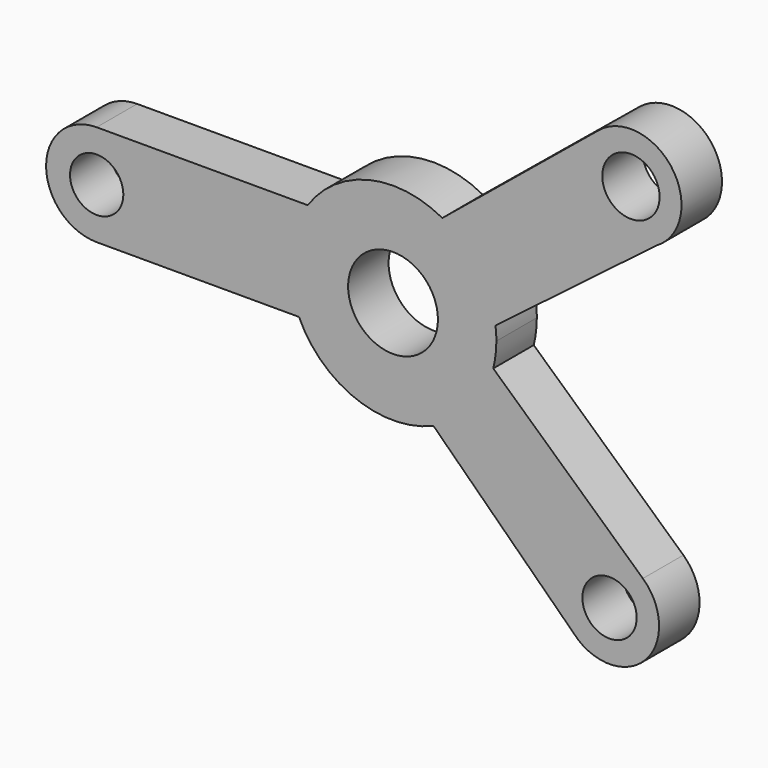
from build123d import *

# Parameters (mm, degrees)
F1_DEPTH  = 25.4
F2_R      = 22.5453784596
F3_DEPTH  = 25.401
F4_R      = 15.5169822629
F4_R_2    = 14.6151483758
F4_R_3    = 13.5851891759
F5_DEPTH  = 419
F6_R      = 14.3828522328
F7_DEPTH  = 25.401
F8_R      = 13.6217726984
F9_DEPTH  = 25.4
F10_R     = 13.3826357349
F11_DEPTH = 25.4


# Not quite as in the source:
# - an extrude ends at something that could not be found from the text; its depth is read off the source's solid


with BuildPart() as f1:
    # F0 (on Front) → F1 (new body)
    with BuildSketch(Plane.XZ):
        with BuildLine():
            ThreePointArc((50.3233435561, -12.5877974986), (51.4847298632, -6.3414622483), (51.873804107, 0))
            ThreePointArc((51.873804107, 0), (51.7629612184, 3.3893064834), (51.4309062461, 6.7641285647))
            ThreePointArc((51.4309062461, 6.7641285647), (42.7546046022, 29.3757610599), (24.7585971482, 45.5840259278))
            ThreePointArc((24.7585971482, 45.5840259278), (-12.1730496974, 50.4252755431), (-42.8284505735, 29.2679923125))
            ThreePointArc((-42.8284505735, 29.2679923125), (-51.683323237, 4.4413569672), (-47.1939000029, -21.5320076875))
            ThreePointArc((-47.1939000029, -21.5320076875), (-18.7719046051, -48.3581135905), (20.3057196076, -47.7343618764))
            ThreePointArc((20.3057196076, -47.7343618764), (39.4453595209, -33.6890956364), (50.3233435561, -12.5877974986))
        make_face()
        with BuildLine():
            ThreePointArc((24.7585971482, 45.5840259278), (42.7546046022, 29.3757610599), (51.4309062461, 6.7641285647))
            Line((51.4309062461, 6.7641285647), (132.2230654066, 68.3692177878))
            ThreePointArc((132.2230654066, 68.3692177878), (140.3155469651, 104.8046621717), (103.3515533001, 109.9711926872))
            Line((103.3515533001, 109.9711926872), (24.7585971482, 45.5840259278))
        make_face()
        with BuildLine():
            Line((125.4517560768, -80.9857626154), (50.3233435561, -12.5877974986))
            ThreePointArc((50.3233435561, -12.5877974986), (39.4453595209, -33.6890956364), (20.3057196076, -47.7343618764))
            Line((20.3057196076, -47.7343618764), (93.0013113713, -118.7126045859))
            ThreePointArc((93.0013113713, -118.7126045859), (127.5656184462, -115.6234022642), (125.4517560768, -80.9857626154))
        make_face()
        with BuildLine():
            ThreePointArc((-47.1939000029, -21.5320076875), (-51.683323237, 4.4413569672), (-42.8284505735, 29.2679923125))
            Line((-42.8284505735, 29.2679923125), (-148.7939000029, 29.2679923125))
            ThreePointArc((-148.7939000029, 29.2679923125), (-174.1939000029, 3.8679923125), (-148.7939000029, -21.5320076875))
            Line((-148.7939000029, -21.5320076875), (-47.1939000029, -21.5320076875))
        make_face()
    extrude(amount=F1_DEPTH)

    # F2 (on face) → F3 (cut, through all)
    with BuildSketch(Plane.XZ.offset(25.4)):
        Circle(F2_R)
    extrude(amount=-F3_DEPTH, mode=Mode.SUBTRACT)

    # F4 (on face) → F5 (cut, through all)
    with BuildSketch(Plane.XZ.offset(25.4)):
        with Locations((119.4483449899, 90.3229536493)):
            Circle(F4_R)
        with Locations((108.694701762, -99.3917325452)):
            Circle(F4_R_2)
        with Locations((-148.7939000029, 3.8679923125)):
            Circle(F4_R_3)
    extrude(amount=F5_DEPTH, mode=Mode.SUBTRACT)

    # F6 (on face) → F7 (cut, through all)
    with BuildSketch(Plane.XZ.offset(25.4)):
        with Locations((119.4483449899, 90.3229536493)):
            Circle(F6_R)
    extrude(amount=-F7_DEPTH, mode=Mode.SUBTRACT)

    # F8 (on face) → F9 (cut)
    with BuildSketch(Plane.XZ.offset(25.4)):
        with Locations((108.694701762, -99.3917325452)):
            Circle(F8_R)
    extrude(amount=-F9_DEPTH, mode=Mode.SUBTRACT)

    # F10 (on face) → F11 (cut)
    with BuildSketch(Plane.XZ.offset(25.4)):
        with Locations((-148.7939000029, 3.8679923125)):
            Circle(F10_R)
    extrude(amount=-F11_DEPTH, mode=Mode.SUBTRACT)


solid = f1.part
